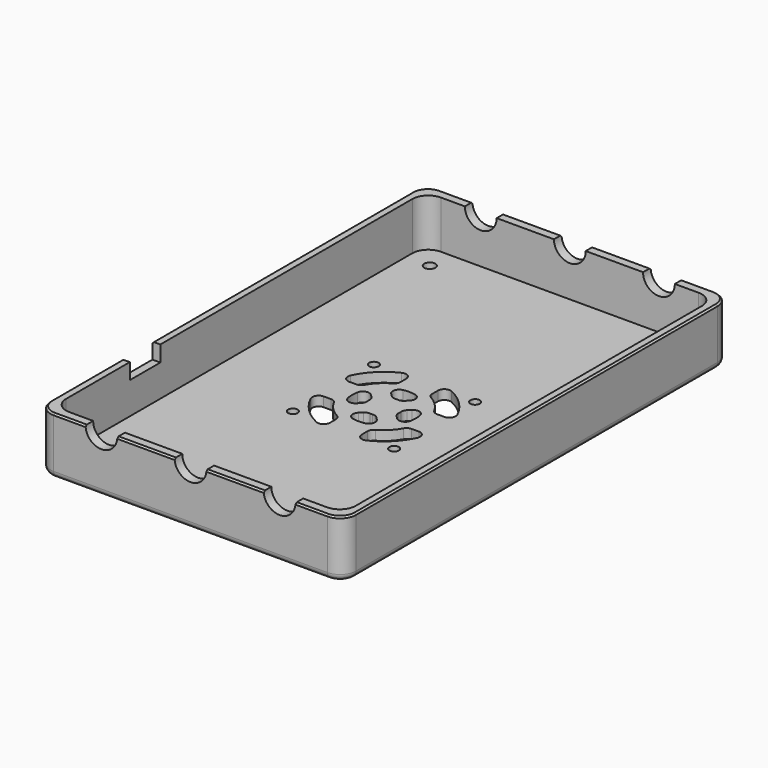
from build123d import *

# Parameters (mm, degrees)
F0_W        = 96
F0_H        = 152
F1_DEPTH    = 3
F2_W        = 96
F2_H        = 152
F2_W_2      = 91
F2_H_2      = 146
F3_DEPTH    = 15
F4_R        = 1.75
F5_DEPTH    = 3
F6_R        = 5
F7_R        = 2
F8_R        = 5
F9_DEPTH    = 152.001
F10_W       = 12
F10_H       = 20.9038736373
F11_DEPTH   = 93.501
F12_R       = 1.5
F13_DEPTH   = 3
F14_C1_SIZE = 0.5
F14_C2_SIZE = 0.5
F14_C3_SIZE = 0.5
F14_C4_SIZE = 0.5
F14_C5_SIZE = 0.5
F14_C6_SIZE = 0.5
F14_C7_SIZE = 0.5


with BuildPart() as f1:
    # F0 (on Top) → F1 (new body)
    with BuildSketch(Plane.XY):
        Rectangle(F0_W, F0_H)
    extrude(amount=F1_DEPTH)

    # F2 (on face) → F3 (join)
    with BuildSketch(Plane.XY.offset(3)):
        Rectangle(F2_W, F2_H)
        Rectangle(F2_W_2, F2_H_2, mode=Mode.SUBTRACT)
    extrude(amount=F3_DEPTH)

    # F4 (on face) → F5 (cut, through all)
    with BuildSketch(Plane.XY.offset(3)):
        with Locations((-38, 65.5)):
            Circle(F4_R)
        with Locations((38, 65.5)):
            Circle(F4_R)
        with Locations((-38, -65.5)):
            Circle(F4_R)
        with Locations((38, -65.5)):
            Circle(F4_R)
    extrude(amount=-F5_DEPTH, mode=Mode.SUBTRACT)

    # F6
    f6_edges = [f1.edges().sort_by_distance(p)[0] for p in [
        (-48, -76, 9),
        (48, -76, 9),
        (45.5, -73, 10.5),
        (-45.5, -73, 10.5),
        (-48, 76, 9),
        (-45.5, 73, 10.5),
        (48, 76, 9),
        (45.5, 73, 10.5),
    ]]
    fillet(f6_edges, radius=F6_R)

    # F7
    f7_edges = [f1.edges().sort_by_distance(p)[0] for p in [
        (-48, 0, 0),
    ]]
    fillet(f7_edges, radius=F7_R)

    # F8 (on face) → F9 (cut, through all)
    with BuildSketch(Plane.XZ.offset(76)):
        with Locations((-28, 18)):
            Circle(F8_R)
        with Locations((0, 18)):
            Circle(F8_R)
        with Locations((28, 18)):
            Circle(F8_R)
    extrude(amount=-F9_DEPTH, mode=Mode.SUBTRACT)

    # F10 (on face) → F11 (cut, through all)
    with BuildSketch(Plane(origin=(45.5, 0, 0), x_dir=(0, -1, 0), z_dir=(-1, 0, 0))):
        with Locations((37, 23.4519368187)):
            Rectangle(F10_W, F10_H)
    extrude(amount=F11_DEPTH, mode=Mode.SUBTRACT)

    # F12 (on face) → F13 (cut, through all)
    with BuildSketch(Plane.XY.offset(3)):
        with Locations((-15.9099025767, -15.9099025767)):
            Circle(F12_R)
        with Locations((15.9099025767, -15.9099025767)):
            Circle(F12_R)
        with Locations((15.9099025767, 15.9099025767)):
            Circle(F12_R)
        with Locations((-15.9099025767, 15.9099025767)):
            Circle(F12_R)
        with BuildLine():
            ThreePointArc((14.9415527975, 5), (16.6292982903, 5.92691326), (16.7526501063, 7.8484848485))
            ThreePointArc((16.7526501063, 7.8484848485), (13.081475452, 13.081475452), (7.8484848485, 16.7526501063))
            ThreePointArc((7.8484848485, 16.7526501063), (5.92691326, 16.6292982903), (5, 14.9415527975))
            Line((5, 14.9415527975), (5, 12.6984250992))
            ThreePointArc((5, 12.6984250992), (5.2779322774, 11.6813298438), (6.0344827586, 10.946918189))
            ThreePointArc((6.0344827586, 10.946918189), (8.8388347648, 8.8388347648), (10.946918189, 6.0344827586))
            ThreePointArc((10.946918189, 6.0344827586), (11.6813298438, 5.2779322774), (12.6984250992, 5))
            Line((12.6984250992, 5), (14.9415527975, 5))
        make_face()
        with BuildLine():
            Line((14.9415527975, -5), (12.6984250992, -5))
            ThreePointArc((12.6984250992, -5), (11.6813298438, -5.2779322774), (10.946918189, -6.0344827586))
            ThreePointArc((10.946918189, -6.0344827586), (8.8388347648, -8.8388347648), (6.0344827586, -10.946918189))
            ThreePointArc((6.0344827586, -10.946918189), (5.2779322774, -11.6813298438), (5, -12.6984250992))
            Line((5, -12.6984250992), (5, -14.9415527975))
            ThreePointArc((5, -14.9415527975), (5.92691326, -16.6292982903), (7.8484848485, -16.7526501063))
            ThreePointArc((7.8484848485, -16.7526501063), (13.081475452, -13.081475452), (16.7526501063, -7.8484848485))
            ThreePointArc((16.7526501063, -7.8484848485), (16.6292982903, -5.92691326), (14.9415527975, -5))
        make_face()
        with BuildLine():
            ThreePointArc((-10.946918189, 6.0344827586), (-8.8388347648, 8.8388347648), (-6.0344827586, 10.946918189))
            ThreePointArc((-6.0344827586, 10.946918189), (-5.2779322774, 11.6813298438), (-5, 12.6984250992))
            Line((-5, 12.6984250992), (-5, 14.9415527975))
            ThreePointArc((-5, 14.9415527975), (-5.92691326, 16.6292982903), (-7.8484848485, 16.7526501063))
            ThreePointArc((-7.8484848485, 16.7526501063), (-13.081475452, 13.081475452), (-16.7526501063, 7.8484848485))
            ThreePointArc((-16.7526501063, 7.8484848485), (-16.6292982903, 5.92691326), (-14.9415527975, 5))
            Line((-14.9415527975, 5), (-12.6984250992, 5))
            ThreePointArc((-12.6984250992, 5), (-11.6813298438, 5.2779322774), (-10.946918189, 6.0344827586))
        make_face()
        with BuildLine():
            ThreePointArc((-6.0344827586, -10.946918189), (-8.8388347648, -8.8388347648), (-10.946918189, -6.0344827586))
            ThreePointArc((-10.946918189, -6.0344827586), (-11.6813298438, -5.2779322774), (-12.6984250992, -5))
            Line((-12.6984250992, -5), (-14.9415527975, -5))
            ThreePointArc((-14.9415527975, -5), (-16.6292982903, -5.92691326), (-16.7526501063, -7.8484848485))
            ThreePointArc((-16.7526501063, -7.8484848485), (-13.081475452, -13.081475452), (-7.8484848485, -16.7526501063))
            ThreePointArc((-7.8484848485, -16.7526501063), (-5.92691326, -16.6292982903), (-5, -14.9415527975))
            Line((-5, -14.9415527975), (-5, -12.6984250992))
            ThreePointArc((-5, -12.6984250992), (-5.2779322774, -11.6813298438), (-6.0344827586, -10.946918189))
        make_face()
        with BuildLine():
            ThreePointArc((6.4448386864, -2.9093047805), (8.447614421, -3.4065290459), (9.823815311, -1.8688640227))
            ThreePointArc((9.823815311, -1.8688640227), (10, 0), (9.823815311, 1.8688640227))
            ThreePointArc((9.823815311, 1.8688640227), (8.447614421, 3.4065290459), (6.4448386864, 2.9093047805))
            Line((6.4448386864, 2.9093047805), (5.559204675, 2.0236707691))
            ThreePointArc((5.559204675, 2.0236707691), (5.0940640438, 1.2935827909), (4.9810130267, 0.4353265762))
            ThreePointArc((4.9810130267, 0.4353265762), (5, 0), (4.9810130267, -0.4353265762))
            ThreePointArc((4.9810130267, -0.4353265762), (5.0940640438, -1.2935827909), (5.559204675, -2.0236707691))
            Line((5.559204675, -2.0236707691), (6.4448386864, -2.9093047805))
        make_face()
        with BuildLine():
            Line((2.9093047805, -6.4448386864), (2.0236707691, -5.559204675))
            ThreePointArc((2.0236707691, -5.559204675), (1.2935827909, -5.0940640438), (0.4353265762, -4.9810130267))
            ThreePointArc((0.4353265762, -4.9810130267), (0, -5), (-0.4353265762, -4.9810130267))
            ThreePointArc((-0.4353265762, -4.9810130267), (-1.2935827909, -5.0940640438), (-2.0236707691, -5.559204675))
            Line((-2.0236707691, -5.559204675), (-2.9093047805, -6.4448386864))
            ThreePointArc((-2.9093047805, -6.4448386864), (-3.4065290459, -8.447614421), (-1.8688640227, -9.823815311))
            ThreePointArc((-1.8688640227, -9.823815311), (0, -10), (1.8688640227, -9.823815311))
            ThreePointArc((1.8688640227, -9.823815311), (3.4065290459, -8.447614421), (2.9093047805, -6.4448386864))
        make_face()
        with BuildLine():
            ThreePointArc((-0.4353265762, 4.9810130267), (0, 5), (0.4353265762, 4.9810130267))
            ThreePointArc((0.4353265762, 4.9810130267), (1.2935827909, 5.0940640438), (2.0236707691, 5.559204675))
            Line((2.0236707691, 5.559204675), (2.9093047805, 6.4448386864))
            ThreePointArc((2.9093047805, 6.4448386864), (3.4065290459, 8.447614421), (1.8688640227, 9.823815311))
            ThreePointArc((1.8688640227, 9.823815311), (0, 10), (-1.8688640227, 9.823815311))
            ThreePointArc((-1.8688640227, 9.823815311), (-3.4065290459, 8.447614421), (-2.9093047805, 6.4448386864))
            Line((-2.9093047805, 6.4448386864), (-2.0236707691, 5.559204675))
            ThreePointArc((-2.0236707691, 5.559204675), (-1.2935827909, 5.0940640438), (-0.4353265762, 4.9810130267))
        make_face()
        with BuildLine():
            ThreePointArc((-4.9810130267, -0.4353265762), (-5, 0), (-4.9810130267, 0.4353265762))
            ThreePointArc((-4.9810130267, 0.4353265762), (-5.0940640438, 1.2935827909), (-5.559204675, 2.0236707691))
            Line((-5.559204675, 2.0236707691), (-6.4448386864, 2.9093047805))
            ThreePointArc((-6.4448386864, 2.9093047805), (-8.447614421, 3.4065290459), (-9.823815311, 1.8688640227))
            ThreePointArc((-9.823815311, 1.8688640227), (-10, 0), (-9.823815311, -1.8688640227))
            ThreePointArc((-9.823815311, -1.8688640227), (-8.447614421, -3.4065290459), (-6.4448386864, -2.9093047805))
            Line((-6.4448386864, -2.9093047805), (-5.559204675, -2.0236707691))
            ThreePointArc((-5.559204675, -2.0236707691), (-5.0940640438, -1.2935827909), (-4.9810130267, -0.4353265762))
        make_face()
    extrude(amount=-F13_DEPTH, mode=Mode.SUBTRACT)

    # F14: chamfer of 0.5 on 7 edges, made by hand

    # F14_c1
    f14_c1_edges = [f1.edges().sort_by_distance(p)[0] for p in [
        (38, -76, 18),
        (46.5355339059, -74.5355339059, 18),
        (48, 0, 18),
        (46.5355339059, 74.5355339059, 18),
        (38, 76, 18),
    ]]
    chamfer(f14_c1_edges, length=F14_C1_SIZE)

    # F14_c2
    f14_c2_edges = [f1.edges().sort_by_distance(p)[0] for p in [
        (14, -76, 18),
    ]]
    chamfer(f14_c2_edges, length=F14_C2_SIZE)

    # F14_c3
    f14_c3_edges = [f1.edges().sort_by_distance(p)[0] for p in [
        (-14, -76, 18),
    ]]
    chamfer(f14_c3_edges, length=F14_C3_SIZE)

    # F14_c4
    f14_c4_edges = [f1.edges().sort_by_distance(p)[0] for p in [
        (-38, -76, 18),
        (-46.5355339059, -74.5355339059, 18),
        (-48, -57, 18),
    ]]
    chamfer(f14_c4_edges, length=F14_C4_SIZE)

    # F14_c5
    f14_c5_edges = [f1.edges().sort_by_distance(p)[0] for p in [
        (-38, 76, 18),
        (-48, 20, 18),
        (-46.5355339059, 74.5355339059, 18),
    ]]
    chamfer(f14_c5_edges, length=F14_C5_SIZE)

    # F14_c6
    f14_c6_edges = [f1.edges().sort_by_distance(p)[0] for p in [
        (-14, 76, 18),
    ]]
    chamfer(f14_c6_edges, length=F14_C6_SIZE)

    # F14_c7
    f14_c7_edges = [f1.edges().sort_by_distance(p)[0] for p in [
        (14, 76, 18),
    ]]
    chamfer(f14_c7_edges, length=F14_C7_SIZE)


solid = f1.part
